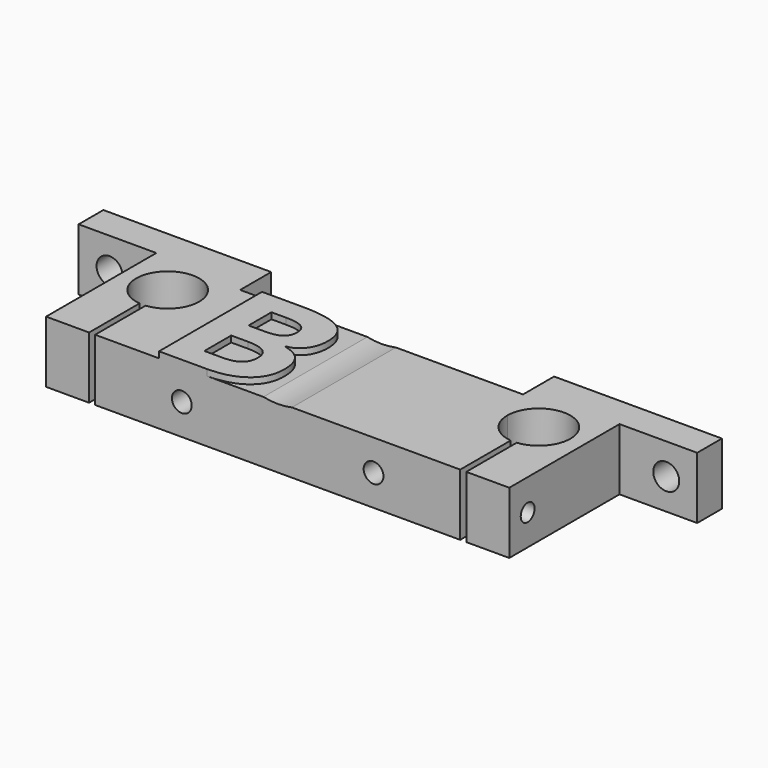
from build123d import *

# Parameters (mm, degrees)
F1_DEPTH      = 10
F2_R          = 1.6
F2_R_2        = 10.75
F3_DEPTH      = 27.2759499461
F4_R          = 2.1
F5_DEPTH      = 5.001
F7_DEPTH      = 10.001
F8_R          = 1.4
F9_DEPTH      = 18
F11_TEXT_SIZE = 29.1666666667
F12_DEPTH     = 1
F8_R_2        = 1.7
F13_DEPTH     = 6.9528983364


# Not quite as in the source:
# - Text() gives the source's letters only with a copy of the font that has no kerning and outlines rounded to 1/6400 em; it was checked with that copy


with BuildPart() as f1:
    # F0 (on Top) → F1 (new body)
    with BuildSketch(Plane.XY):
        Polygon((-37.4418646097, -13.8158900663), (0, -13.8158900663), (0, 7.1841099337), (-22.8655805642, 7.1841099337), (-22.8655805642, 13.4590598798), (-50, 13.4590598798), (-50, 8.4590598798), (-37.4418646097, 8.4590598798), align=None)
    extrude(amount=F1_DEPTH)

    # F2 (on face) → F3 (cut, through all)
    with BuildSketch(Plane.XZ.offset(13.8158900663)):
        with Locations((-15.5, 5)):
            Circle(F2_R)
        with Locations((0, 20.5)):
            Circle(F2_R_2)
    extrude(amount=-F3_DEPTH, mode=Mode.SUBTRACT)

    # F4 (on face) → F5 (cut, through all)
    with BuildSketch(Plane.XZ.offset(-8.4590598798)):
        with Locations((-45, 5)):
            Circle(F4_R)
    extrude(amount=-F5_DEPTH, mode=Mode.SUBTRACT)

    # F6 (on face) → F7 (cut, through all)
    with BuildSketch(Plane.XY.offset(10)):
        with BuildLine():
            ThreePointArc((-29.5100337267, -3.6173495847), (-26.2244981795, -1.9695821259), (-24.9, 1.4590598798))
            ThreePointArc((-24.9, 1.4590598798), (-33.4286420057, 5.2345617004), (-30.4899662733, -3.6173495847))
            Line((-30.4899662733, -3.6173495847), (-30.4899662733, -2.0438153297))
            Line((-30.4899662733, -2.0438153297), (-29.5100337267, -2.0438153297))
            Line((-29.5100337267, -2.0438153297), (-29.5100337267, -3.6173495847))
        make_face()
        with BuildLine():
            Line((-30.4899662733, -2.0438153297), (-30.4899662733, -3.6173495847))
            ThreePointArc((-30.4899662733, -3.6173495847), (-30, -3.6409401202), (-29.5100337267, -3.6173495847))
            Line((-29.5100337267, -3.6173495847), (-29.5100337267, -2.0438153297))
            Line((-29.5100337267, -2.0438153297), (-30.4899662733, -2.0438153297))
        make_face()
        with BuildLine():
            ThreePointArc((-29.5100337267, -3.6173495847), (-30, -3.6409401202), (-30.4899662733, -3.6173495847))
            Line((-30.4899662733, -3.6173495847), (-30.4899662733, -14.1640976071))
            Line((-30.4899662733, -14.1640976071), (-29.5100337267, -14.1640976071))
            Line((-29.5100337267, -14.1640976071), (-29.5100337267, -3.6173495847))
        make_face()
    extrude(amount=-F7_DEPTH, mode=Mode.SUBTRACT)

    # F8 (on face) → F9 (cut)
    with BuildSketch(Plane(origin=(-37.4418646097, 0, 0), x_dir=(0, -1, 0), z_dir=(-1, 0, 0))):
        with Locations((10.1014729589, 4.9766320735)):
            Circle(F8_R)
    extrude(amount=-F9_DEPTH, mode=Mode.SUBTRACT)

    # F10: F1 across plane


with BuildPart() as f1_1:
    add(f1.part)
    add(f1.part.mirror(Plane.YZ))

    # F11 (on face) → F12 (join)
    with BuildSketch(Plane.XY.offset(10)):
        with Locations((-21.8066685395, -13.8158900663)):
            Text('B', F11_TEXT_SIZE, font='Open Sans', font_style=FontStyle.BOLD, text_align=(TextAlign.LEFT, TextAlign.BOTTOM))
    extrude(amount=F12_DEPTH)

    # F8 (on face) → F13 (cut, through all)
    with BuildSketch(Plane(origin=(-37.4418646097, 0, 0), x_dir=(0, -1, 0), z_dir=(-1, 0, 0))):
        with Locations((10.1014729589, 4.9766320735)):
            Circle(F8_R_2)
        with Locations((10.1014729589, 4.9766320735)):
            Circle(F8_R, mode=Mode.SUBTRACT)
        with Locations((10.1014729589, 4.9766320735)):
            Circle(F8_R)
    extrude(amount=-F13_DEPTH, mode=Mode.SUBTRACT)


solid = f1_1.part
